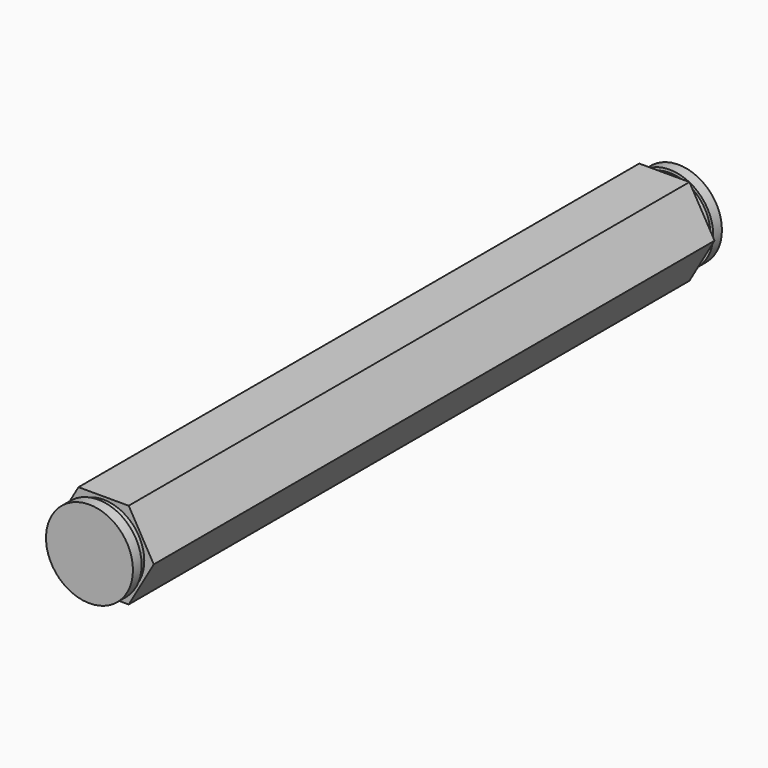
from build123d import *

# Parameters (mm, degrees)
F1_DEPTH      = 51.196875
F1_DEPTH_BACK = 51.196875
F2_R          = 5.9436
F3_DEPTH      = 0.9906
F4_R          = 6.35
F5_DEPTH      = 1.5875


# Not quite as in the source:
# - a pattern or mirror of a feature is missing from the dataset's text; its kind, count and spacing are read off the source's solid


with BuildPart() as f1:
    # F0 (on Front) → F1 (new body, two sides)
    with BuildSketch(Plane.XZ) as f1_sk:
        Polygon((3.6661742094, 6.35), (-3.6661742094, 6.35), (-7.3323484187, 0), (-3.6661742094, -6.35), (3.6661742094, -6.35), (7.3323484187, 0), align=None)
    extrude(amount=F1_DEPTH)
    extrude(f1_sk.sketch, amount=-F1_DEPTH_BACK)

    # F2 (on face) → F3 (join)
    with BuildSketch(Plane.XZ.offset(51.196875)):
        Circle(F2_R)
    f3 = extrude(amount=F3_DEPTH)

    # F3_copies: F3 across plane
    add(f3.mirror(Plane.ZX))

    # F4 (on face) → F5 (join)
    with BuildSketch(Plane.XZ.offset(52.187475)):
        Circle(F4_R)
    f5 = extrude(amount=F5_DEPTH)

    # F5_copies: F5 across plane
    add(f5.mirror(Plane.ZX))


solid = f1.part
